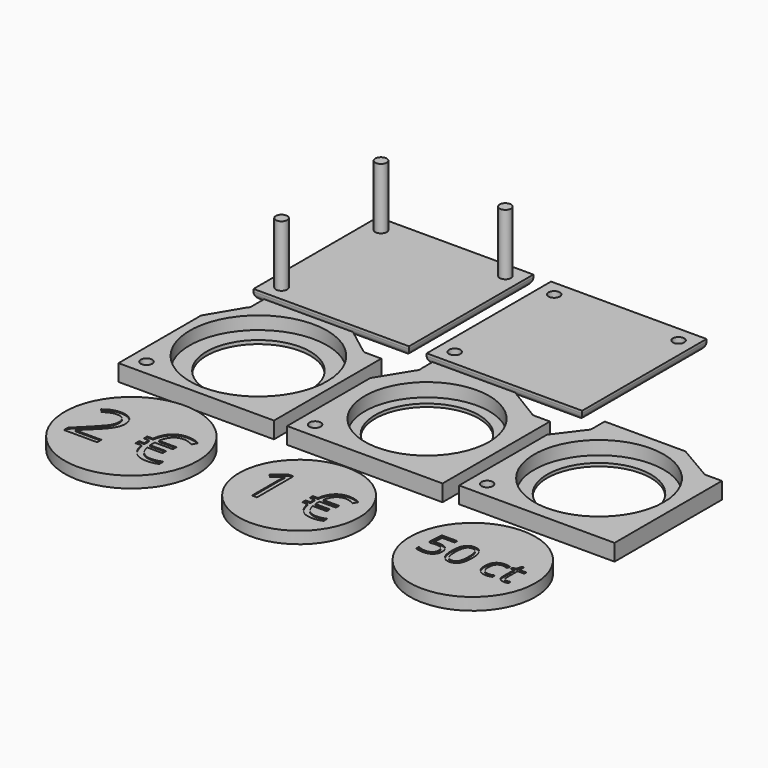
from build123d import *

# Parameters (mm, degrees)
F0_R            = 1.1
F1_DEPTH        = 13.8
F0_W            = 30
F0_H            = 30
F2_DEPTH        = 2
F3_R            = 1.1
F4_DEPTH        = 0.2
F3_W            = 30
F3_H            = 30
F5_DEPTH        = 2
F6_R            = 1.5
F6_2_R          = 1.5
F7_R            = 1.1
F7_R_2          = 13.25
F8_DEPTH        = 3.2
F7_R_3          = 10
F9_DEPTH        = 0.7
F10_R           = 1.1
F10_R_2         = 12
F10_R_3         = 10
F11_DEPTH       = 0.6
F12_DEPTH       = 3.2
F13_R           = 12.5
F13_R_2         = 10
F14_DEPTH       = 0.6
F13_R_3         = 1.1
F15_DEPTH       = 3.2
F16_R           = 12.85
F17_DEPTH       = 2.2
F16_R_2         = 11.6
F16_R_3         = 12.1
F16_TEXT_SIZE   = 13.6679124399
F18_DEPTH       = 2
F19_DEPTH       = 2.3
F16_TEXT_SIZE_2 = 12.3011211959
F20_DEPTH       = 2.1
F21_DEPTH       = 2.35
F16_TEXT_SIZE_3 = 8.3470620538
F22_DEPTH       = 2.15


# Not quite as in the source:
# - Text() gives the source's letters only with a copy of the font that has no kerning and outlines rounded to 1/6400 em; it was checked with that copy


with BuildPart() as f1:
    # F0 (on Top) → F1 (new body)
    with BuildSketch(Plane.XY):
        with Locations((-44.7898054395, 43.5211111382)):
            Circle(F0_R)
    extrude(amount=F1_DEPTH)


with BuildPart() as f1b:
    # F0 (on Top) → F1, piece 2 (new body)
    with BuildSketch(Plane.XY):
        with Locations((-20.7898054395, 43.5211111382)):
            Circle(F0_R)
    extrude(amount=F1_DEPTH)


with BuildPart() as f1c:
    # F0 (on Top) → F1, piece 3 (new body)
    with BuildSketch(Plane.XY):
        with Locations((-44.7898054395, 19.5211111382)):
            Circle(F0_R)
    extrude(amount=F1_DEPTH)


with BuildPart() as f2:
    # F0 (on Top) → F2 (new body)
    with BuildSketch(Plane.XY):
        with Locations((-32.7898054395, 31.5211111382)):
            Rectangle(F0_W, F0_H)
        with Locations((-44.7898054395, 19.5211111382)):
            Circle(F0_R, mode=Mode.SUBTRACT)
        with Locations((-44.7898054395, 43.5211111382)):
            Circle(F0_R, mode=Mode.SUBTRACT)
        with Locations((-20.7898054395, 43.5211111382)):
            Circle(F0_R, mode=Mode.SUBTRACT)
    extrude(amount=F2_DEPTH)

    # F6
    f6_edges = [f2.edges().sort_by_distance(p)[0] for p in [
        (-47.789805, 31.521111, 0),
        (-32.789805, 46.521111, 0),
        (-17.789805, 31.521111, 0),
        (-32.789805, 16.521111, 0),
    ]]
    fillet(f6_edges, radius=F6_R)


with BuildPart() as f4:
    # F3 (on Top) → F4 (new body)
    with BuildSketch(Plane.XY):
        with Locations((-11.2770004198, 43.4070006013)):
            Circle(F3_R)
    extrude(amount=F4_DEPTH)


with BuildPart() as f4b:
    # F3 (on Top) → F4, piece 2 (new body)
    with BuildSketch(Plane.XY):
        with Locations((12.7229995802, 43.4070006013)):
            Circle(F3_R)
    extrude(amount=F4_DEPTH)


with BuildPart() as f4c:
    # F3 (on Top) → F4, piece 3 (new body)
    with BuildSketch(Plane.XY):
        with Locations((-11.2770004198, 19.4070006013)):
            Circle(F3_R)
    extrude(amount=F4_DEPTH)


with BuildPart() as f5:
    # F3 (on Top) → F5 (new body)
    with BuildSketch(Plane.XY):
        with Locations((0.7229995802, 31.4070006013)):
            Rectangle(F3_W, F3_H)
        with Locations((-11.2770004198, 19.4070006013)):
            Circle(F3_R, mode=Mode.SUBTRACT)
        with Locations((-11.2770004198, 43.4070006013)):
            Circle(F3_R, mode=Mode.SUBTRACT)
        with Locations((12.7229995802, 43.4070006013)):
            Circle(F3_R, mode=Mode.SUBTRACT)
    extrude(amount=F5_DEPTH)

    # F6#2
    f6_2_edges = [f5.edges().sort_by_distance(p)[0] for p in [
        (-14.277, 31.407001, 0),
        (0.723, 46.407001, 0),
        (15.723, 31.407001, 0),
        (0.723, 16.407001, 0),
    ]]
    fillet(f6_2_edges, radius=F6_2_R)


with BuildPart() as f8:
    # F7 (on Top) → F8 (new body)
    with BuildSketch(Plane.XY):
        with BuildLine():
            Line((-25.8606971163, 13.0906781201), (-43.0029673813, 13.0906781201))
            Line((-43.0029673813, 13.0906781201), (-43.0029673813, 10.0906781201))
            ThreePointArc((-43.0029673813, 10.0906781201), (-43.1021662122, 9.6341728957), (-43.3818710539, 9.2600036432))
            Line((-43.3818710539, 9.2600036432), (-47.1029673813, 2.9990995356))
            Line((-47.1029673813, 2.9990995356), (-47.1029673813, -16.9093218799))
            Line((-47.1029673813, -16.9093218799), (-17.1029673813, -16.9093218799))
            Line((-17.1029673813, -16.9093218799), (-17.1029673813, 8.9906781201))
            Line((-17.1029673813, 8.9906781201), (-20.1029673813, 8.9906781201))
            ThreePointArc((-20.1029673813, 8.9906781201), (-20.4939169, 9.0624959992), (-20.8338170274, 9.2685718041))
            Line((-20.8338170274, 9.2685718041), (-25.8606971163, 13.0906781201))
        make_face()
        with Locations((-44.1029673813, -13.9093218799)):
            Circle(F7_R, mode=Mode.SUBTRACT)
        with Locations((-32.1029673813, -1.9093218799)):
            Circle(F7_R_2, mode=Mode.SUBTRACT)
    extrude(amount=F8_DEPTH)

    # F7 (on Top) → F9 (join)
    with BuildSketch(Plane.XY):
        with Locations((-32.1029673813, -1.9093218799)):
            Circle(F7_R_2)
        with Locations((-32.1029673813, -1.9093218799)):
            Circle(F7_R_3, mode=Mode.SUBTRACT)
    extrude(amount=F9_DEPTH)


with BuildPart() as f11:
    # F10 (on Top) → F11 (new body)
    with BuildSketch(Plane.XY):
        with BuildLine():
            Line((5.5624246375, 12.928437885), (-10.368363773, 12.928437885))
            Line((-10.368363773, 12.928437885), (-10.368363773, 10.1843869379))
            ThreePointArc((-10.368363773, 10.1843869379), (-10.3457461724, 10.0572996796), (-10.3381722056, 9.928437885))
            ThreePointArc((-10.3381722056, 9.928437885), (-10.4185691016, 9.5156310168), (-10.6480076791, 9.1631666775))
            Line((-10.6480076791, 9.1631666775), (-14.4381722056, 3.0001146088))
            Line((-14.4381722056, 3.0001146088), (-14.4381722056, -17.071562115))
            Line((-14.4381722056, -17.071562115), (15.5618277944, -17.071562115))
            Line((15.5618277944, -17.071562115), (15.5618277944, 8.828437885))
            Line((15.5618277944, 8.828437885), (12.5618277944, 8.828437885))
            ThreePointArc((12.5618277944, 8.828437885), (12.1555647522, 8.9062097595), (11.8067486887, 9.1285281751))
            Line((11.8067486887, 9.1285281751), (5.5624246375, 12.928437885))
        make_face()
        with Locations((-11.4381722056, -14.071562115)):
            Circle(F10_R, mode=Mode.SUBTRACT)
        with Locations((0.5618277944, -2.071562115)):
            Circle(F10_R_2, mode=Mode.SUBTRACT)
        with Locations((0.5618277944, -2.071562115)):
            Circle(F10_R_2)
        with Locations((0.5618277944, -2.071562115)):
            Circle(F10_R_3, mode=Mode.SUBTRACT)
    extrude(amount=F11_DEPTH)

    # F10 (on Top) → F12 (join)
    with BuildSketch(Plane.XY):
        with BuildLine():
            Line((5.5624246375, 12.928437885), (-10.368363773, 12.928437885))
            Line((-10.368363773, 12.928437885), (-10.368363773, 10.1843869379))
            ThreePointArc((-10.368363773, 10.1843869379), (-10.3457461724, 10.0572996796), (-10.3381722056, 9.928437885))
            ThreePointArc((-10.3381722056, 9.928437885), (-10.4185691016, 9.5156310168), (-10.6480076791, 9.1631666775))
            Line((-10.6480076791, 9.1631666775), (-14.4381722056, 3.0001146088))
            Line((-14.4381722056, 3.0001146088), (-14.4381722056, -17.071562115))
            Line((-14.4381722056, -17.071562115), (15.5618277944, -17.071562115))
            Line((15.5618277944, -17.071562115), (15.5618277944, 8.828437885))
            Line((15.5618277944, 8.828437885), (12.5618277944, 8.828437885))
            ThreePointArc((12.5618277944, 8.828437885), (12.1555647522, 8.9062097595), (11.8067486887, 9.1285281751))
            Line((11.8067486887, 9.1285281751), (5.5624246375, 12.928437885))
        make_face()
        with Locations((-11.4381722056, -14.071562115)):
            Circle(F10_R, mode=Mode.SUBTRACT)
        with Locations((0.5618277944, -2.071562115)):
            Circle(F10_R_2, mode=Mode.SUBTRACT)
    extrude(amount=F12_DEPTH)


with BuildPart() as f14:
    # F13 (on Top) → F14 (new body)
    with BuildSketch(Plane.XY):
        with Locations((32.917368561, -1.0191252171)):
            Circle(F13_R)
        with Locations((32.917368561, -1.0191252171)):
            Circle(F13_R_2, mode=Mode.SUBTRACT)
    extrude(amount=F14_DEPTH)

    # F13 (on Top) → F15 (join)
    with BuildSketch(Plane.XY):
        with BuildLine():
            Line((37.5873016656, 13.9808747829), (22.017368561, 13.9808747829))
            Line((22.017368561, 13.9808747829), (22.017368561, 10.9808747829))
            ThreePointArc((22.017368561, 10.9808747829), (21.9220451909, 10.5329631071), (21.6525960714, 10.1626813412))
            Line((21.6525960714, 10.1626813412), (17.917368561, 5.2009611391))
            Line((17.917368561, 5.2009611391), (17.917368561, -16.0191252171))
            Line((17.917368561, -16.0191252171), (47.917368561, -16.0191252171))
            Line((47.917368561, -16.0191252171), (47.917368561, 9.8808747829))
            Line((47.917368561, 9.8808747829), (44.917368561, 9.8808747829))
            ThreePointArc((44.917368561, 9.8808747829), (44.6060378321, 9.9258519503), (44.3201666929, 10.0571053697))
            Line((44.3201666929, 10.0571053697), (37.5873016656, 13.9808747829))
        make_face()
        with Locations((20.917368561, -13.0191252171)):
            Circle(F13_R_3, mode=Mode.SUBTRACT)
        with Locations((32.917368561, -1.0191252171)):
            Circle(F13_R, mode=Mode.SUBTRACT)
    extrude(amount=F15_DEPTH)


with BuildPart() as f17:
    # F16 (on Top) → F17 (new body)
    with BuildSketch(Plane.XY):
        with Locations((-31.8807428401, -32.8427363563)):
            Circle(F16_R)
        with BuildLine():
            Line((-34.6803298381, -36.5603660624), (-34.6803298381, -37.5875951067))
            Line((-34.6803298381, -37.5875951067), (-41.0935706283, -37.5875951067))
            Line((-41.0935706283, -37.5875951067), (-41.0935706283, -36.6329768472))
            Line((-41.0935706283, -36.6329768472), (-38.5244302119, -34.0510227629))
            add(Edge.make_bspline(
                [(-38.5244302119, -34.0510227629), (-37.3498439866, -32.8614872583), (-36.9761120058, -32.3542795701)],
                knots=[0, 0, 0, 1, 1, 1], degree=2))
            add(Edge.make_bspline(
                [(-36.9761120058, -32.3542795701), (-36.602380025, -31.8470718819), (-36.4155140346, -31.3665593352)],
                knots=[0, 0, 0, 1, 1, 1], degree=2))
            add(Edge.make_bspline(
                [(-36.4155140346, -31.3665593352), (-36.2286480442, -30.8860467885), (-36.2286480442, -30.3329234569)],
                knots=[0, 0, 0, 1, 1, 1], degree=2))
            add(Edge.make_bspline(
                [(-36.2286480442, -30.3329234569), (-36.2286480442, -29.5512897143), (-36.702753757, -29.0942688921)],
                knots=[0, 0, 0, 1, 1, 1], degree=2))
            add(Edge.make_bspline(
                [(-36.702753757, -29.0942688921), (-37.1768594697, -28.6372480698), (-38.0182903293, -28.6372480698)],
                knots=[0, 0, 0, 1, 1, 1], degree=2))
            add(Edge.make_bspline(
                [(-38.0182903293, -28.6372480698), (-38.6248039438, -28.6372480698), (-39.1693848301, -28.8379955338)],
                knots=[0, 0, 0, 1, 1, 1], degree=2))
            add(Edge.make_bspline(
                [(-39.1693848301, -28.8379955338), (-39.7139657164, -29.0387429978), (-40.3802764479, -29.5662389935)],
                knots=[0, 0, 0, 1, 1, 1], degree=2))
            Line((-40.3802764479, -29.5662389935), (-40.9675695605, -28.812368198))
            add(Edge.make_bspline(
                [(-40.9675695605, -28.812368198), (-39.6199988184, -27.6911722556), (-38.0311039972, -27.6911722556)],
                knots=[0, 0, 0, 1, 1, 1], degree=2))
            add(Edge.make_bspline(
                [(-38.0311039972, -27.6911722556), (-36.655770308, -27.6911722556), (-35.875204371, -28.3948561852)],
                knots=[0, 0, 0, 1, 1, 1], degree=2))
            add(Edge.make_bspline(
                [(-35.875204371, -28.3948561852), (-35.094638434, -29.0985401147), (-35.094638434, -30.2859400079)],
                knots=[0, 0, 0, 1, 1, 1], degree=2))
            add(Edge.make_bspline(
                [(-35.094638434, -30.2859400079), (-35.094638434, -31.2149309316), (-35.6157275957, -32.122565742)],
                knots=[0, 0, 0, 1, 1, 1], degree=2))
            add(Edge.make_bspline(
                [(-35.6157275957, -32.122565742), (-36.1368167575, -33.0302005525), (-37.5634051184, -34.4183479097)],
                knots=[0, 0, 0, 1, 1, 1], degree=2))
            Line((-37.5634051184, -34.4183479097), (-39.6990164372, -36.5069757794))
            Line((-39.6990164372, -36.5069757794), (-39.6990164372, -36.5603660624))
            Line((-39.6990164372, -36.5603660624), (-34.6803298381, -36.5603660624))
        make_face(mode=Mode.SUBTRACT)
        with BuildLine():
            add(Edge.make_bspline(
                [(-23.1224013811, -29.2651177976), (-24.2286480442, -28.6906383528), (-25.091435017, -28.6906383528)],
                knots=[0, 0, 0, 1, 1, 1], degree=2))
            add(Edge.make_bspline(
                [(-25.091435017, -28.6906383528), (-27.2185038905, -28.6906383528), (-27.7459998862, -31.3815086144)],
                knots=[0, 0, 0, 1, 1, 1], degree=2))
            Line((-27.7459998862, -31.3815086144), (-24.3439710554, -31.3815086144))
            Line((-24.3439710554, -31.3815086144), (-24.3439710554, -32.2421599759))
            Line((-24.3439710554, -32.2421599759), (-27.8399667842, -32.2421599759))
            Line((-27.8399667842, -32.2421599759), (-27.8527804521, -32.6222987906))
            Line((-27.8527804521, -32.6222987906), (-27.8527804521, -33.0494210544))
            Line((-27.8527804521, -33.0494210544), (-27.8399667842, -33.3505422503))
            Line((-27.8399667842, -33.3505422503), (-24.749737206, -33.3505422503))
            Line((-24.749737206, -33.3505422503), (-24.749737206, -34.2111936118))
            Line((-24.749737206, -34.2111936118), (-27.7331862183, -34.2111936118))
            add(Edge.make_bspline(
                [(-27.7331862183, -34.2111936118), (-27.4854553053, -35.4114071729), (-26.8084665173, -36.0691754591)],
                knots=[0, 0, 0, 1, 1, 1], degree=2))
            add(Edge.make_bspline(
                [(-26.8084665173, -36.0691754591), (-26.1314777292, -36.7269437452), (-24.997468119, -36.7269437452)],
                knots=[0, 0, 0, 1, 1, 1], degree=2))
            add(Edge.make_bspline(
                [(-24.997468119, -36.7269437452), (-23.9552897954, -36.7269437452), (-22.9344675851, -36.2870078136)],
                knots=[0, 0, 0, 1, 1, 1], degree=2))
            Line((-22.9344675851, -36.2870078136), (-22.9344675851, -37.2864739107))
            add(Edge.make_bspline(
                [(-22.9344675851, -37.2864739107), (-23.9083063464, -37.7221386198), (-25.0508584019, -37.7221386198)],
                knots=[0, 0, 0, 1, 1, 1], degree=2))
            add(Edge.make_bspline(
                [(-25.0508584019, -37.7221386198), (-26.6312107778, -37.7221386198), (-27.5965070939, -36.8241140602)],
                knots=[0, 0, 0, 1, 1, 1], degree=2))
            add(Edge.make_bspline(
                [(-27.5965070939, -36.8241140602), (-28.5618034099, -35.9260895007), (-28.8671958285, -34.2111936118)],
                knots=[0, 0, 0, 1, 1, 1], degree=2))
            Line((-28.8671958285, -34.2111936118), (-29.9755781029, -34.2111936118))
            Line((-29.9755781029, -34.2111936118), (-29.9755781029, -33.3505422503))
            Line((-29.9755781029, -33.3505422503), (-28.9611627265, -33.3505422503))
            Line((-28.9611627265, -33.3505422503), (-28.9739763945, -33.0686415562))
            Line((-28.9739763945, -33.0686415562), (-28.9739763945, -32.7760628056))
            Line((-28.9739763945, -32.7760628056), (-28.9611627265, -32.2421599759))
            Line((-28.9611627265, -32.2421599759), (-29.9755781029, -32.2421599759))
            Line((-29.9755781029, -32.2421599759), (-29.9755781029, -31.3815086144))
            Line((-29.9755781029, -31.3815086144), (-28.8821451078, -31.3815086144))
            add(Edge.make_bspline(
                [(-28.8821451078, -31.3815086144), (-28.6216005269, -29.6388497783), (-27.6466939599, -28.665011017)],
                knots=[0, 0, 0, 1, 1, 1], degree=2))
            add(Edge.make_bspline(
                [(-27.6466939599, -28.665011017), (-26.6717873929, -27.6911722556), (-25.091435017, -27.6911722556)],
                knots=[0, 0, 0, 1, 1, 1], degree=2))
            add(Edge.make_bspline(
                [(-25.091435017, -27.6911722556), (-23.7481354975, -27.6911722556), (-22.6482956684, -28.3382624852)],
                knots=[0, 0, 0, 1, 1, 1], degree=2))
            Line((-22.6482956684, -28.3382624852), (-23.1224013811, -29.2651177976))
        make_face(mode=Mode.SUBTRACT)
    extrude(amount=F17_DEPTH)

    # F16 (on Top) → F18 (join)
    with BuildSketch(Plane.XY):
        with Locations((-41.7620169711, -37.5875951067)):
            Text('2 €', F16_TEXT_SIZE, font='Open Sans', text_align=(TextAlign.LEFT, TextAlign.BOTTOM))
    extrude(amount=F18_DEPTH)


with BuildPart() as f17b:
    # F16 (on Top) → F17, piece 2 (new body)
    with BuildSketch(Plane.XY):
        with Locations((0, -32.2289278704)):
            Circle(F16_R_2)
        with BuildLine():
            Line((-4.5175740633, -27.9545189204), (-4.5175740633, -36.7363662242))
            Line((-4.5175740633, -36.7363662242), (-5.4901314578, -36.7363662242))
            Line((-5.4901314578, -36.7363662242), (-5.4901314578, -30.4781708157))
            add(Edge.make_bspline(
                [(-5.4901314578, -30.4781708157), (-5.4901314578, -29.6958963897), (-5.4420802031, -29.000114222)],
                knots=[0, 0, 0, 1, 1, 1], degree=2))
            add(Edge.make_bspline(
                [(-5.4420802031, -29.000114222), (-5.5670134653, -29.1269695344), (-5.7236605555, -29.2643961227)],
                knots=[0, 0, 0, 1, 1, 1], degree=2))
            add(Edge.make_bspline(
                [(-5.7236605555, -29.2643961227), (-5.8803076457, -29.4018227111), (-7.1527048694, -30.4358857116)],
                knots=[0, 0, 0, 1, 1, 1], degree=2))
            Line((-7.1527048694, -30.4358857116), (-7.6812686708, -29.7516358451))
            Line((-7.6812686708, -29.7516358451), (-5.3575099949, -27.9545189204))
            Line((-5.3575099949, -27.9545189204), (-4.5175740633, -27.9545189204))
        make_face(mode=Mode.SUBTRACT)
        with BuildLine():
            add(Edge.make_bspline(
                [(7.9642198503, -29.2461366459), (6.9685978535, -28.7291051457), (6.192089578, -28.7291051457)],
                knots=[0, 0, 0, 1, 1, 1], degree=2))
            add(Edge.make_bspline(
                [(6.192089578, -28.7291051457), (4.2777275918, -28.7291051457), (3.8029811957, -31.1508883811)],
                knots=[0, 0, 0, 1, 1, 1], degree=2))
            Line((3.8029811957, -31.1508883811), (6.8648071434, -31.1508883811))
            Line((6.8648071434, -31.1508883811), (6.8648071434, -31.9254746064))
            Line((6.8648071434, -31.9254746064), (3.7184109875, -31.9254746064))
            Line((3.7184109875, -31.9254746064), (3.7068786863, -32.2675995397))
            Line((3.7068786863, -32.2675995397), (3.7068786863, -32.6520095771))
            Line((3.7068786863, -32.6520095771), (3.7184109875, -32.9230186534))
            Line((3.7184109875, -32.9230186534), (6.4996176079, -32.9230186534))
            Line((6.4996176079, -32.9230186534), (6.4996176079, -33.6976048787))
            Line((6.4996176079, -33.6976048787), (3.8145134968, -33.6976048787))
            add(Edge.make_bspline(
                [(3.8145134968, -33.6976048787), (4.0374713185, -34.7777970837), (4.6467612277, -35.3697885413)],
                knots=[0, 0, 0, 1, 1, 1], degree=2))
            add(Edge.make_bspline(
                [(4.6467612277, -35.3697885413), (5.256051137, -35.9617799989), (6.2766597862, -35.9617799989)],
                knots=[0, 0, 0, 1, 1, 1], degree=2))
            add(Edge.make_bspline(
                [(6.2766597862, -35.9617799989), (7.2146202774, -35.9617799989), (8.1333602667, -35.5658376604)],
                knots=[0, 0, 0, 1, 1, 1], degree=2))
            Line((8.1333602667, -35.5658376604), (8.1333602667, -36.4653571478))
            add(Edge.make_bspline(
                [(8.1333602667, -36.4653571478), (7.2569053815, -36.8574553859), (6.2286085315, -36.8574553859)],
                knots=[0, 0, 0, 1, 1, 1], degree=2))
            add(Edge.make_bspline(
                [(6.2286085315, -36.8574553859), (4.8062913932, -36.8574553859), (3.9375247088, -36.0492332824)],
                knots=[0, 0, 0, 1, 1, 1], degree=2))
            add(Edge.make_bspline(
                [(3.9375247088, -36.0492332824), (3.0687580243, -35.2410111788), (2.7939048476, -33.6976048787)],
                knots=[0, 0, 0, 1, 1, 1], degree=2))
            Line((2.7939048476, -33.6976048787), (1.7963608006, -33.6976048787))
            Line((1.7963608006, -33.6976048787), (1.7963608006, -32.9230186534))
            Line((1.7963608006, -32.9230186534), (2.7093346394, -32.9230186534))
            Line((2.7093346394, -32.9230186534), (2.6978023382, -32.6693080288))
            Line((2.6978023382, -32.6693080288), (2.6978023382, -32.4059871532))
            Line((2.6978023382, -32.4059871532), (2.7093346394, -31.9254746064))
            Line((2.7093346394, -31.9254746064), (1.7963608006, -31.9254746064))
            Line((1.7963608006, -31.9254746064), (1.7963608006, -31.1508883811))
            Line((1.7963608006, -31.1508883811), (2.7804504963, -31.1508883811))
            add(Edge.make_bspline(
                [(2.7804504963, -31.1508883811), (3.0149406191, -29.5824954286), (3.8923565294, -28.7060405434)],
                knots=[0, 0, 0, 1, 1, 1], degree=2))
            add(Edge.make_bspline(
                [(3.8923565294, -28.7060405434), (4.7697724397, -27.8295856582), (6.192089578, -27.8295856582)],
                knots=[0, 0, 0, 1, 1, 1], degree=2))
            add(Edge.make_bspline(
                [(6.192089578, -27.8295856582), (7.4010591455, -27.8295856582), (8.3909149917, -28.4119668648)],
                knots=[0, 0, 0, 1, 1, 1], degree=2))
            Line((8.3909149917, -28.4119668648), (7.9642198503, -29.2461366459))
        make_face(mode=Mode.SUBTRACT)
    extrude(amount=F17_DEPTH)

    # F16 (on Top) → F19 (join)
    with BuildSketch(Plane.XY):
        with Locations((0, -32.2289278704)):
            Circle(F16_R_2)
        with BuildLine():
            Line((-4.5175740633, -27.9545189204), (-4.5175740633, -36.7363662242))
            Line((-4.5175740633, -36.7363662242), (-5.4901314578, -36.7363662242))
            Line((-5.4901314578, -36.7363662242), (-5.4901314578, -30.4781708157))
            add(Edge.make_bspline(
                [(-5.4901314578, -30.4781708157), (-5.4901314578, -29.6958963897), (-5.4420802031, -29.000114222)],
                knots=[0, 0, 0, 1, 1, 1], degree=2))
            add(Edge.make_bspline(
                [(-5.4420802031, -29.000114222), (-5.5670134653, -29.1269695344), (-5.7236605555, -29.2643961227)],
                knots=[0, 0, 0, 1, 1, 1], degree=2))
            add(Edge.make_bspline(
                [(-5.7236605555, -29.2643961227), (-5.8803076457, -29.4018227111), (-7.1527048694, -30.4358857116)],
                knots=[0, 0, 0, 1, 1, 1], degree=2))
            Line((-7.1527048694, -30.4358857116), (-7.6812686708, -29.7516358451))
            Line((-7.6812686708, -29.7516358451), (-5.3575099949, -27.9545189204))
            Line((-5.3575099949, -27.9545189204), (-4.5175740633, -27.9545189204))
        make_face(mode=Mode.SUBTRACT)
        with BuildLine():
            add(Edge.make_bspline(
                [(7.9642198503, -29.2461366459), (6.9685978535, -28.7291051457), (6.192089578, -28.7291051457)],
                knots=[0, 0, 0, 1, 1, 1], degree=2))
            add(Edge.make_bspline(
                [(6.192089578, -28.7291051457), (4.2777275918, -28.7291051457), (3.8029811957, -31.1508883811)],
                knots=[0, 0, 0, 1, 1, 1], degree=2))
            Line((3.8029811957, -31.1508883811), (6.8648071434, -31.1508883811))
            Line((6.8648071434, -31.1508883811), (6.8648071434, -31.9254746064))
            Line((6.8648071434, -31.9254746064), (3.7184109875, -31.9254746064))
            Line((3.7184109875, -31.9254746064), (3.7068786863, -32.2675995397))
            Line((3.7068786863, -32.2675995397), (3.7068786863, -32.6520095771))
            Line((3.7068786863, -32.6520095771), (3.7184109875, -32.9230186534))
            Line((3.7184109875, -32.9230186534), (6.4996176079, -32.9230186534))
            Line((6.4996176079, -32.9230186534), (6.4996176079, -33.6976048787))
            Line((6.4996176079, -33.6976048787), (3.8145134968, -33.6976048787))
            add(Edge.make_bspline(
                [(3.8145134968, -33.6976048787), (4.0374713185, -34.7777970837), (4.6467612277, -35.3697885413)],
                knots=[0, 0, 0, 1, 1, 1], degree=2))
            add(Edge.make_bspline(
                [(4.6467612277, -35.3697885413), (5.256051137, -35.9617799989), (6.2766597862, -35.9617799989)],
                knots=[0, 0, 0, 1, 1, 1], degree=2))
            add(Edge.make_bspline(
                [(6.2766597862, -35.9617799989), (7.2146202774, -35.9617799989), (8.1333602667, -35.5658376604)],
                knots=[0, 0, 0, 1, 1, 1], degree=2))
            Line((8.1333602667, -35.5658376604), (8.1333602667, -36.4653571478))
            add(Edge.make_bspline(
                [(8.1333602667, -36.4653571478), (7.2569053815, -36.8574553859), (6.2286085315, -36.8574553859)],
                knots=[0, 0, 0, 1, 1, 1], degree=2))
            add(Edge.make_bspline(
                [(6.2286085315, -36.8574553859), (4.8062913932, -36.8574553859), (3.9375247088, -36.0492332824)],
                knots=[0, 0, 0, 1, 1, 1], degree=2))
            add(Edge.make_bspline(
                [(3.9375247088, -36.0492332824), (3.0687580243, -35.2410111788), (2.7939048476, -33.6976048787)],
                knots=[0, 0, 0, 1, 1, 1], degree=2))
            Line((2.7939048476, -33.6976048787), (1.7963608006, -33.6976048787))
            Line((1.7963608006, -33.6976048787), (1.7963608006, -32.9230186534))
            Line((1.7963608006, -32.9230186534), (2.7093346394, -32.9230186534))
            Line((2.7093346394, -32.9230186534), (2.6978023382, -32.6693080288))
            Line((2.6978023382, -32.6693080288), (2.6978023382, -32.4059871532))
            Line((2.6978023382, -32.4059871532), (2.7093346394, -31.9254746064))
            Line((2.7093346394, -31.9254746064), (1.7963608006, -31.9254746064))
            Line((1.7963608006, -31.9254746064), (1.7963608006, -31.1508883811))
            Line((1.7963608006, -31.1508883811), (2.7804504963, -31.1508883811))
            add(Edge.make_bspline(
                [(2.7804504963, -31.1508883811), (3.0149406191, -29.5824954286), (3.8923565294, -28.7060405434)],
                knots=[0, 0, 0, 1, 1, 1], degree=2))
            add(Edge.make_bspline(
                [(3.8923565294, -28.7060405434), (4.7697724397, -27.8295856582), (6.192089578, -27.8295856582)],
                knots=[0, 0, 0, 1, 1, 1], degree=2))
            add(Edge.make_bspline(
                [(6.192089578, -27.8295856582), (7.4010591455, -27.8295856582), (8.3909149917, -28.4119668648)],
                knots=[0, 0, 0, 1, 1, 1], degree=2))
            Line((8.3909149917, -28.4119668648), (7.9642198503, -29.2461366459))
        make_face(mode=Mode.SUBTRACT)
    extrude(amount=F19_DEPTH)

    # F16 (on Top) → F20 (join)
    with BuildSketch(Plane.XY):
        with Locations((-8.8114341807, -36.7363662242)):
            Text('1 €', F16_TEXT_SIZE_2, font='Open Sans', text_align=(TextAlign.LEFT, TextAlign.BOTTOM))
    extrude(amount=F20_DEPTH)


with BuildPart() as f17c:
    # F16 (on Top) → F17, piece 3 (new body)
    with BuildSketch(Plane.XY):
        with Locations((33.6872787919, -32.43638638)):
            Circle(F16_R_3)
        with BuildLine():
            add(Edge.make_bspline(
                [(25.4719588911, -31.500281689), (25.9401769032, -31.4063772409), (26.4057864584, -31.4063772409)],
                knots=[0, 0, 0, 1, 1, 1], degree=2))
            add(Edge.make_bspline(
                [(26.4057864584, -31.4063772409), (27.3474393963, -31.4063772409), (27.8873899729, -31.8732910245)],
                knots=[0, 0, 0, 1, 1, 1], degree=2))
            add(Edge.make_bspline(
                [(27.8873899729, -31.8732910245), (28.4273405495, -32.3402048082), (28.4273405495, -33.1514349015)],
                knots=[0, 0, 0, 1, 1, 1], degree=2))
            add(Edge.make_bspline(
                [(28.4273405495, -33.1514349015), (28.4273405495, -34.0761328697), (27.8384814062, -34.6023890476)],
                knots=[0, 0, 0, 1, 1, 1], degree=2))
            add(Edge.make_bspline(
                [(27.8384814062, -34.6023890476), (27.2496222629, -35.1286452255), (26.2140648768, -35.1286452255)],
                knots=[0, 0, 0, 1, 1, 1], degree=2))
            add(Edge.make_bspline(
                [(26.2140648768, -35.1286452255), (25.2072005166, -35.1286452255), (24.6776837676, -34.8065007994)],
                knots=[0, 0, 0, 1, 1, 1], degree=2))
            Line((24.6776837676, -34.8065007994), (24.6776837676, -34.1543865764))
            add(Edge.make_bspline(
                [(24.6776837676, -34.1543865764), (24.9620055688, -34.3369785589), (25.3858798137, -34.4413168345)],
                knots=[0, 0, 0, 1, 1, 1], degree=2))
            add(Edge.make_bspline(
                [(25.3858798137, -34.4413168345), (25.8097540586, -34.5456551102), (26.2218902475, -34.5456551102)],
                knots=[0, 0, 0, 1, 1, 1], degree=2))
            add(Edge.make_bspline(
                [(26.2218902475, -34.5456551102), (26.9392158928, -34.5456551102), (27.3363534545, -34.2072078285)],
                knots=[0, 0, 0, 1, 1, 1], degree=2))
            add(Edge.make_bspline(
                [(27.3363534545, -34.2072078285), (27.7334910163, -33.8687605468), (27.7334910163, -33.2283843798)],
                knots=[0, 0, 0, 1, 1, 1], degree=2))
            add(Edge.make_bspline(
                [(27.7334910163, -33.2283843798), (27.7334910163, -31.9815419856), (26.2062395062, -31.9815419856)],
                knots=[0, 0, 0, 1, 1, 1], degree=2))
            add(Edge.make_bspline(
                [(26.2062395062, -31.9815419856), (25.8188836577, -31.9815419856), (25.1706821201, -32.1002267741)],
                knots=[0, 0, 0, 1, 1, 1], degree=2))
            Line((25.1706821201, -32.1002267741), (24.8198446682, -31.8758994814))
            Line((24.8198446682, -31.8758994814), (25.0441719609, -29.0874590641))
            Line((25.0441719609, -29.0874590641), (28.00737899, -29.0874590641))
            Line((28.00737899, -29.0874590641), (28.00737899, -29.7108802612))
            Line((28.00737899, -29.7108802612), (25.6232493908, -29.7108802612))
            Line((25.6232493908, -29.7108802612), (25.4719588911, -31.500281689))
        make_face(mode=Mode.SUBTRACT)
        with BuildLine():
            add(Edge.make_bspline(
                [(32.7612916753, -29.7806564831), (33.2647238554, -30.5677583502), (33.2647238554, -32.0584914639)],
                knots=[0, 0, 0, 1, 1, 1], degree=2))
            add(Edge.make_bspline(
                [(33.2647238554, -32.0584914639), (33.2647238554, -33.6040021723), (32.7775945309, -34.3663236989)],
                knots=[0, 0, 0, 1, 1, 1], degree=2))
            add(Edge.make_bspline(
                [(32.7775945309, -34.3663236989), (32.2904652063, -35.1286452255), (31.2875135314, -35.1286452255)],
                knots=[0, 0, 0, 1, 1, 1], degree=2))
            add(Edge.make_bspline(
                [(31.2875135314, -35.1286452255), (30.3262971668, -35.1286452255), (29.8248213293, -34.3480645007)],
                knots=[0, 0, 0, 1, 1, 1], degree=2))
            add(Edge.make_bspline(
                [(29.8248213293, -34.3480645007), (29.3233454919, -33.5674837758), (29.3233454919, -32.0584914639)],
                knots=[0, 0, 0, 1, 1, 1], degree=2))
            add(Edge.make_bspline(
                [(29.3233454919, -32.0584914639), (29.3233454919, -30.5025469279), (29.8085184738, -29.7480507719)],
                knots=[0, 0, 0, 1, 1, 1], degree=2))
            add(Edge.make_bspline(
                [(29.8085184738, -29.7480507719), (30.2936914556, -28.993554616), (31.2875135314, -28.993554616)],
                knots=[0, 0, 0, 1, 1, 1], degree=2))
            add(Edge.make_bspline(
                [(31.2875135314, -28.993554616), (32.2578594952, -28.993554616), (32.7612916753, -29.7806564831)],
                knots=[0, 0, 0, 1, 1, 1], degree=2))
        make_face(mode=Mode.SUBTRACT)
        with BuildLine():
            add(Edge.make_bspline(
                [(39.4793724002, -34.8951883337), (39.0320220432, -35.1286452255), (38.3512147945, -35.1286452255)],
                knots=[0, 0, 0, 1, 1, 1], degree=2))
            add(Edge.make_bspline(
                [(38.3512147945, -35.1286452255), (37.3808688307, -35.1286452255), (36.8487436248, -34.5313085973)],
                knots=[0, 0, 0, 1, 1, 1], degree=2))
            add(Edge.make_bspline(
                [(36.8487436248, -34.5313085973), (36.3166184188, -33.9339719691), (36.3166184188, -32.8410285314)],
                knots=[0, 0, 0, 1, 1, 1], degree=2))
            add(Edge.make_bspline(
                [(36.3166184188, -32.8410285314), (36.3166184188, -31.7206962964), (36.8572211097, -31.1090131552)],
                knots=[0, 0, 0, 1, 1, 1], degree=2))
            add(Edge.make_bspline(
                [(36.8572211097, -31.1090131552), (37.3978238005, -30.4973300141), (38.3955585616, -30.4973300141)],
                knots=[0, 0, 0, 1, 1, 1], degree=2))
            add(Edge.make_bspline(
                [(38.3955585616, -30.4973300141), (38.7177029878, -30.4973300141), (39.0398474139, -30.567106236)],
                knots=[0, 0, 0, 1, 1, 1], degree=2))
            add(Edge.make_bspline(
                [(39.0398474139, -30.567106236), (39.36199184, -30.6368824578), (39.5445838225, -30.7307869059)],
                knots=[0, 0, 0, 1, 1, 1], degree=2))
            Line((39.5445838225, -30.7307869059), (39.3372114996, -31.3046474221))
            add(Edge.make_bspline(
                [(39.3372114996, -31.3046474221), (39.1128842069, -31.2146556594), (38.8481258324, -31.1559653793)],
                knots=[0, 0, 0, 1, 1, 1], degree=2))
            add(Edge.make_bspline(
                [(38.8481258324, -31.1559653793), (38.5833674578, -31.0972750992), (38.3799078203, -31.0972750992)],
                knots=[0, 0, 0, 1, 1, 1], degree=2))
            add(Edge.make_bspline(
                [(38.3799078203, -31.0972750992), (37.0182933227, -31.0972750992), (37.0182933227, -32.8332031607)],
                knots=[0, 0, 0, 1, 1, 1], degree=2))
            add(Edge.make_bspline(
                [(37.0182933227, -32.8332031607), (37.0182933227, -33.6561713101), (37.3502194622, -34.0963484106)],
                knots=[0, 0, 0, 1, 1, 1], degree=2))
            add(Edge.make_bspline(
                [(37.3502194622, -34.0963484106), (37.6821456017, -34.5365255111), (38.3342598247, -34.5365255111)],
                knots=[0, 0, 0, 1, 1, 1], degree=2))
            add(Edge.make_bspline(
                [(38.3342598247, -34.5365255111), (38.8924695995, -34.5365255111), (39.4793724002, -34.296547477)],
                knots=[0, 0, 0, 1, 1, 1], degree=2))
            Line((39.4793724002, -34.296547477), (39.4793724002, -34.8951883337))
        make_face(mode=Mode.SUBTRACT)
        with BuildLine():
            add(Edge.make_bspline(
                [(41.4565827242, -34.3532814144), (41.6483043057, -34.5691312222), (41.9821867879, -34.5691312222)],
                knots=[0, 0, 0, 1, 1, 1], degree=2))
            add(Edge.make_bspline(
                [(41.9821867879, -34.5691312222), (42.1621703134, -34.5691312222), (42.3291115545, -34.5430466533)],
                knots=[0, 0, 0, 1, 1, 1], degree=2))
            add(Edge.make_bspline(
                [(42.3291115545, -34.5430466533), (42.4960527956, -34.5169620844), (42.593869929, -34.4882690586)],
                knots=[0, 0, 0, 1, 1, 1], degree=2))
            Line((42.593869929, -34.4882690586), (42.593869929, -35.0060477516))
            add(Edge.make_bspline(
                [(42.593869929, -35.0060477516), (42.4843147396, -35.0582168895), (42.2704212744, -35.0934310575)],
                knots=[0, 0, 0, 1, 1, 1], degree=2))
            add(Edge.make_bspline(
                [(42.2704212744, -35.0934310575), (42.0565278093, -35.1286452255), (41.8843696544, -35.1286452255)],
                knots=[0, 0, 0, 1, 1, 1], degree=2))
            add(Edge.make_bspline(
                [(41.8843696544, -35.1286452255), (40.5892708076, -35.1286452255), (40.5892708076, -33.7631180427)],
                knots=[0, 0, 0, 1, 1, 1], degree=2))
            Line((40.5892708076, -33.7631180427), (40.5892708076, -31.1051004699))
            Line((40.5892708076, -31.1051004699), (39.9488946407, -31.1051004699))
            Line((39.9488946407, -31.1051004699), (39.9488946407, -30.7790433584))
            Line((39.9488946407, -30.7790433584), (40.5892708076, -30.4973300141))
            Line((40.5892708076, -30.4973300141), (40.8735926089, -29.5439390202))
            Line((40.8735926089, -29.5439390202), (41.2648611426, -29.5439390202))
            Line((41.2648611426, -29.5439390202), (41.2648611426, -30.5794964062))
            Line((41.2648611426, -30.5794964062), (42.5612642179, -30.5794964062))
            Line((42.5612642179, -30.5794964062), (42.5612642179, -31.1051004699))
            Line((42.5612642179, -31.1051004699), (41.2648611426, -31.1051004699))
            Line((41.2648611426, -31.1051004699), (41.2648611426, -33.7344250169))
            add(Edge.make_bspline(
                [(41.2648611426, -33.7344250169), (41.2648611426, -34.1374316066), (41.4565827242, -34.3532814144)],
                knots=[0, 0, 0, 1, 1, 1], degree=2))
        make_face(mode=Mode.SUBTRACT)
    extrude(amount=F17_DEPTH)

    # F16 (on Top) → F21 (join)
    with BuildSketch(Plane.XY):
        with Locations((33.6872787919, -32.43638638)):
            Circle(F16_R_3)
        with BuildLine():
            add(Edge.make_bspline(
                [(25.4719588911, -31.500281689), (25.9401769032, -31.4063772409), (26.4057864584, -31.4063772409)],
                knots=[0, 0, 0, 1, 1, 1], degree=2))
            add(Edge.make_bspline(
                [(26.4057864584, -31.4063772409), (27.3474393963, -31.4063772409), (27.8873899729, -31.8732910245)],
                knots=[0, 0, 0, 1, 1, 1], degree=2))
            add(Edge.make_bspline(
                [(27.8873899729, -31.8732910245), (28.4273405495, -32.3402048082), (28.4273405495, -33.1514349015)],
                knots=[0, 0, 0, 1, 1, 1], degree=2))
            add(Edge.make_bspline(
                [(28.4273405495, -33.1514349015), (28.4273405495, -34.0761328697), (27.8384814062, -34.6023890476)],
                knots=[0, 0, 0, 1, 1, 1], degree=2))
            add(Edge.make_bspline(
                [(27.8384814062, -34.6023890476), (27.2496222629, -35.1286452255), (26.2140648768, -35.1286452255)],
                knots=[0, 0, 0, 1, 1, 1], degree=2))
            add(Edge.make_bspline(
                [(26.2140648768, -35.1286452255), (25.2072005166, -35.1286452255), (24.6776837676, -34.8065007994)],
                knots=[0, 0, 0, 1, 1, 1], degree=2))
            Line((24.6776837676, -34.8065007994), (24.6776837676, -34.1543865764))
            add(Edge.make_bspline(
                [(24.6776837676, -34.1543865764), (24.9620055688, -34.3369785589), (25.3858798137, -34.4413168345)],
                knots=[0, 0, 0, 1, 1, 1], degree=2))
            add(Edge.make_bspline(
                [(25.3858798137, -34.4413168345), (25.8097540586, -34.5456551102), (26.2218902475, -34.5456551102)],
                knots=[0, 0, 0, 1, 1, 1], degree=2))
            add(Edge.make_bspline(
                [(26.2218902475, -34.5456551102), (26.9392158928, -34.5456551102), (27.3363534545, -34.2072078285)],
                knots=[0, 0, 0, 1, 1, 1], degree=2))
            add(Edge.make_bspline(
                [(27.3363534545, -34.2072078285), (27.7334910163, -33.8687605468), (27.7334910163, -33.2283843798)],
                knots=[0, 0, 0, 1, 1, 1], degree=2))
            add(Edge.make_bspline(
                [(27.7334910163, -33.2283843798), (27.7334910163, -31.9815419856), (26.2062395062, -31.9815419856)],
                knots=[0, 0, 0, 1, 1, 1], degree=2))
            add(Edge.make_bspline(
                [(26.2062395062, -31.9815419856), (25.8188836577, -31.9815419856), (25.1706821201, -32.1002267741)],
                knots=[0, 0, 0, 1, 1, 1], degree=2))
            Line((25.1706821201, -32.1002267741), (24.8198446682, -31.8758994814))
            Line((24.8198446682, -31.8758994814), (25.0441719609, -29.0874590641))
            Line((25.0441719609, -29.0874590641), (28.00737899, -29.0874590641))
            Line((28.00737899, -29.0874590641), (28.00737899, -29.7108802612))
            Line((28.00737899, -29.7108802612), (25.6232493908, -29.7108802612))
            Line((25.6232493908, -29.7108802612), (25.4719588911, -31.500281689))
        make_face(mode=Mode.SUBTRACT)
        with BuildLine():
            add(Edge.make_bspline(
                [(32.7612916753, -29.7806564831), (33.2647238554, -30.5677583502), (33.2647238554, -32.0584914639)],
                knots=[0, 0, 0, 1, 1, 1], degree=2))
            add(Edge.make_bspline(
                [(33.2647238554, -32.0584914639), (33.2647238554, -33.6040021723), (32.7775945309, -34.3663236989)],
                knots=[0, 0, 0, 1, 1, 1], degree=2))
            add(Edge.make_bspline(
                [(32.7775945309, -34.3663236989), (32.2904652063, -35.1286452255), (31.2875135314, -35.1286452255)],
                knots=[0, 0, 0, 1, 1, 1], degree=2))
            add(Edge.make_bspline(
                [(31.2875135314, -35.1286452255), (30.3262971668, -35.1286452255), (29.8248213293, -34.3480645007)],
                knots=[0, 0, 0, 1, 1, 1], degree=2))
            add(Edge.make_bspline(
                [(29.8248213293, -34.3480645007), (29.3233454919, -33.5674837758), (29.3233454919, -32.0584914639)],
                knots=[0, 0, 0, 1, 1, 1], degree=2))
            add(Edge.make_bspline(
                [(29.3233454919, -32.0584914639), (29.3233454919, -30.5025469279), (29.8085184738, -29.7480507719)],
                knots=[0, 0, 0, 1, 1, 1], degree=2))
            add(Edge.make_bspline(
                [(29.8085184738, -29.7480507719), (30.2936914556, -28.993554616), (31.2875135314, -28.993554616)],
                knots=[0, 0, 0, 1, 1, 1], degree=2))
            add(Edge.make_bspline(
                [(31.2875135314, -28.993554616), (32.2578594952, -28.993554616), (32.7612916753, -29.7806564831)],
                knots=[0, 0, 0, 1, 1, 1], degree=2))
        make_face(mode=Mode.SUBTRACT)
        with BuildLine():
            add(Edge.make_bspline(
                [(39.4793724002, -34.8951883337), (39.0320220432, -35.1286452255), (38.3512147945, -35.1286452255)],
                knots=[0, 0, 0, 1, 1, 1], degree=2))
            add(Edge.make_bspline(
                [(38.3512147945, -35.1286452255), (37.3808688307, -35.1286452255), (36.8487436248, -34.5313085973)],
                knots=[0, 0, 0, 1, 1, 1], degree=2))
            add(Edge.make_bspline(
                [(36.8487436248, -34.5313085973), (36.3166184188, -33.9339719691), (36.3166184188, -32.8410285314)],
                knots=[0, 0, 0, 1, 1, 1], degree=2))
            add(Edge.make_bspline(
                [(36.3166184188, -32.8410285314), (36.3166184188, -31.7206962964), (36.8572211097, -31.1090131552)],
                knots=[0, 0, 0, 1, 1, 1], degree=2))
            add(Edge.make_bspline(
                [(36.8572211097, -31.1090131552), (37.3978238005, -30.4973300141), (38.3955585616, -30.4973300141)],
                knots=[0, 0, 0, 1, 1, 1], degree=2))
            add(Edge.make_bspline(
                [(38.3955585616, -30.4973300141), (38.7177029878, -30.4973300141), (39.0398474139, -30.567106236)],
                knots=[0, 0, 0, 1, 1, 1], degree=2))
            add(Edge.make_bspline(
                [(39.0398474139, -30.567106236), (39.36199184, -30.6368824578), (39.5445838225, -30.7307869059)],
                knots=[0, 0, 0, 1, 1, 1], degree=2))
            Line((39.5445838225, -30.7307869059), (39.3372114996, -31.3046474221))
            add(Edge.make_bspline(
                [(39.3372114996, -31.3046474221), (39.1128842069, -31.2146556594), (38.8481258324, -31.1559653793)],
                knots=[0, 0, 0, 1, 1, 1], degree=2))
            add(Edge.make_bspline(
                [(38.8481258324, -31.1559653793), (38.5833674578, -31.0972750992), (38.3799078203, -31.0972750992)],
                knots=[0, 0, 0, 1, 1, 1], degree=2))
            add(Edge.make_bspline(
                [(38.3799078203, -31.0972750992), (37.0182933227, -31.0972750992), (37.0182933227, -32.8332031607)],
                knots=[0, 0, 0, 1, 1, 1], degree=2))
            add(Edge.make_bspline(
                [(37.0182933227, -32.8332031607), (37.0182933227, -33.6561713101), (37.3502194622, -34.0963484106)],
                knots=[0, 0, 0, 1, 1, 1], degree=2))
            add(Edge.make_bspline(
                [(37.3502194622, -34.0963484106), (37.6821456017, -34.5365255111), (38.3342598247, -34.5365255111)],
                knots=[0, 0, 0, 1, 1, 1], degree=2))
            add(Edge.make_bspline(
                [(38.3342598247, -34.5365255111), (38.8924695995, -34.5365255111), (39.4793724002, -34.296547477)],
                knots=[0, 0, 0, 1, 1, 1], degree=2))
            Line((39.4793724002, -34.296547477), (39.4793724002, -34.8951883337))
        make_face(mode=Mode.SUBTRACT)
        with BuildLine():
            add(Edge.make_bspline(
                [(41.4565827242, -34.3532814144), (41.6483043057, -34.5691312222), (41.9821867879, -34.5691312222)],
                knots=[0, 0, 0, 1, 1, 1], degree=2))
            add(Edge.make_bspline(
                [(41.9821867879, -34.5691312222), (42.1621703134, -34.5691312222), (42.3291115545, -34.5430466533)],
                knots=[0, 0, 0, 1, 1, 1], degree=2))
            add(Edge.make_bspline(
                [(42.3291115545, -34.5430466533), (42.4960527956, -34.5169620844), (42.593869929, -34.4882690586)],
                knots=[0, 0, 0, 1, 1, 1], degree=2))
            Line((42.593869929, -34.4882690586), (42.593869929, -35.0060477516))
            add(Edge.make_bspline(
                [(42.593869929, -35.0060477516), (42.4843147396, -35.0582168895), (42.2704212744, -35.0934310575)],
                knots=[0, 0, 0, 1, 1, 1], degree=2))
            add(Edge.make_bspline(
                [(42.2704212744, -35.0934310575), (42.0565278093, -35.1286452255), (41.8843696544, -35.1286452255)],
                knots=[0, 0, 0, 1, 1, 1], degree=2))
            add(Edge.make_bspline(
                [(41.8843696544, -35.1286452255), (40.5892708076, -35.1286452255), (40.5892708076, -33.7631180427)],
                knots=[0, 0, 0, 1, 1, 1], degree=2))
            Line((40.5892708076, -33.7631180427), (40.5892708076, -31.1051004699))
            Line((40.5892708076, -31.1051004699), (39.9488946407, -31.1051004699))
            Line((39.9488946407, -31.1051004699), (39.9488946407, -30.7790433584))
            Line((39.9488946407, -30.7790433584), (40.5892708076, -30.4973300141))
            Line((40.5892708076, -30.4973300141), (40.8735926089, -29.5439390202))
            Line((40.8735926089, -29.5439390202), (41.2648611426, -29.5439390202))
            Line((41.2648611426, -29.5439390202), (41.2648611426, -30.5794964062))
            Line((41.2648611426, -30.5794964062), (42.5612642179, -30.5794964062))
            Line((42.5612642179, -30.5794964062), (42.5612642179, -31.1051004699))
            Line((42.5612642179, -31.1051004699), (41.2648611426, -31.1051004699))
            Line((41.2648611426, -31.1051004699), (41.2648611426, -33.7344250169))
            add(Edge.make_bspline(
                [(41.2648611426, -33.7344250169), (41.2648611426, -34.1374316066), (41.4565827242, -34.3532814144)],
                knots=[0, 0, 0, 1, 1, 1], degree=2))
        make_face(mode=Mode.SUBTRACT)
    extrude(amount=F21_DEPTH)


with BuildPart() as f21:
    # F16 (on Top) → F21, piece 2 (new body)
    with BuildSketch(Plane.XY):
        with BuildLine():
            add(Edge.make_bspline(
                [(30.3139069966, -30.16931656), (30.008065426, -30.7581757033), (30.008065426, -32.0584914639)],
                knots=[0, 0, 0, 1, 1, 1], degree=2))
            add(Edge.make_bspline(
                [(30.008065426, -32.0584914639), (30.008065426, -33.3588072244), (30.3139069966, -33.9522311673)],
                knots=[0, 0, 0, 1, 1, 1], degree=2))
            add(Edge.make_bspline(
                [(30.3139069966, -33.9522311673), (30.6197485671, -34.5456551102), (31.2875135314, -34.5456551102)],
                knots=[0, 0, 0, 1, 1, 1], degree=2))
            add(Edge.make_bspline(
                [(31.2875135314, -34.5456551102), (31.9644080949, -34.5456551102), (32.2676412085, -33.9444057966)],
                knots=[0, 0, 0, 1, 1, 1], degree=2))
            add(Edge.make_bspline(
                [(32.2676412085, -33.9444057966), (32.5708743222, -33.3431564831), (32.5708743222, -32.0584914639)],
                knots=[0, 0, 0, 1, 1, 1], degree=2))
            add(Edge.make_bspline(
                [(32.5708743222, -32.0584914639), (32.5708743222, -30.7751306731), (32.2676412085, -30.1777940449)],
                knots=[0, 0, 0, 1, 1, 1], degree=2))
            add(Edge.make_bspline(
                [(32.2676412085, -30.1777940449), (31.9644080949, -29.5804574166), (31.2875135314, -29.5804574166)],
                knots=[0, 0, 0, 1, 1, 1], degree=2))
            add(Edge.make_bspline(
                [(31.2875135314, -29.5804574166), (30.6197485671, -29.5804574166), (30.3139069966, -30.16931656)],
                knots=[0, 0, 0, 1, 1, 1], degree=2))
        make_face()
    extrude(amount=F21_DEPTH)


with BuildPart() as f22:
    # F16 (on Top) → F22 (new body)
    with BuildSketch(Plane.XY):
        with Locations((24.1351247341, -35.0464788334)):
            Text('50 ct', F16_TEXT_SIZE_3, font='Open Sans', text_align=(TextAlign.LEFT, TextAlign.BOTTOM))
    extrude(amount=F22_DEPTH)


solid = Compound([f1.part, f1b.part, f1c.part, f2.part, f4.part, f4b.part, f4c.part, f5.part, f8.part, f11.part, f14.part, f17.part, f17b.part, f17c.part, f21.part, f22.part])
